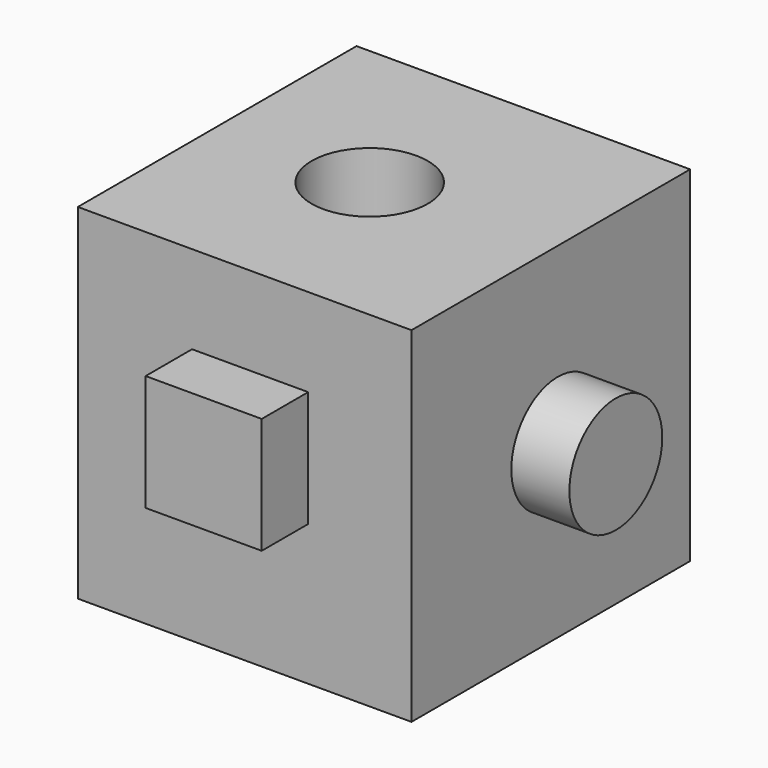
from build123d import *

# Parameters (mm, degrees)
F0_W     = 72.9848642368
F0_H     = 75.440466404
F1_DEPTH = 76.2
F3_D     = 25.4
F4_W     = 25.4
F4_H     = 25.4
F5_DEPTH = 12.7
F7_R     = 12.7
F8_DEPTH = 12.7


# Not quite as in the source:
# - a length typed as a fraction of an inch, garbled in the dataset ("3 / 203.2 mm" for 3/8 in), is restored


with BuildPart() as f1:
    # F0 (on Front) → F1 (new body)
    with BuildSketch(Plane.XZ):
        with Locations((39.7899424424, 37.720233202)):
            Rectangle(F0_W, F0_H)
    extrude(amount=F1_DEPTH)

    # F3 (through all)
    with Locations(Plane.XY.offset(75.440466404)):
        with Locations((36.5493223071, -37.9619333167)):
            Hole(F3_D / 2)

    # F4 (on face) → F5 (join)
    with BuildSketch(Plane.XZ.offset(76.2)):
        with Locations((40.9810889382, 43.4622988105)):
            Rectangle(F4_W, F4_H)
    extrude(amount=F5_DEPTH)

    # F7 (on face) → F8 (join)
    with BuildSketch(Plane.YZ.offset(76.2823745608)):
        with Locations((-36.2048484385, 37.505440414)):
            Circle(F7_R)
    extrude(amount=F8_DEPTH)


solid = f1.part
